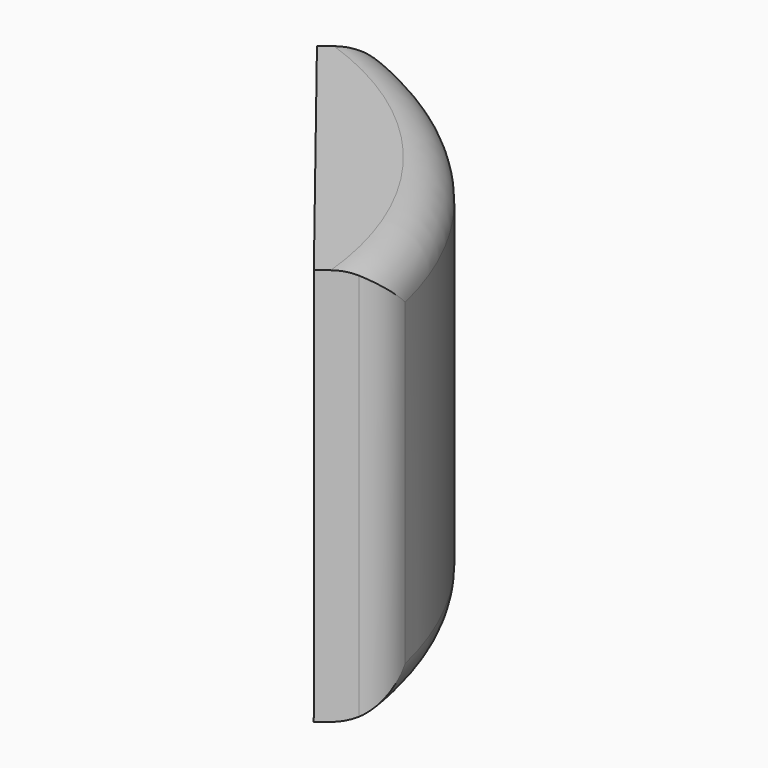
from build123d import *

# Parameters (mm, degrees)
F1_DEPTH     = 50.8
F2_W         = 48.4209248795
F2_H         = 50.8
F2_W_2       = 40.64
F2_H_2       = 40.64
F3_DEPTH     = 7.62
F4_T1_DEPTH  = 40.64
F4_T3_DEPTH  = 40.64
F4_T9_DEPTH  = 53.34
F4_T15_DEPTH = 53.34
F4_T24_DEPTH = 53.34
F4_T30_DEPTH = 53.34
F5_T1_DEPTH  = 40.64
F5_T6_DEPTH  = 17.2700101558
F5_S7_R      = 5.0800000001
F5_T8_DEPTH  = 13
F5_T12_DEPTH = 15.9109147238
F5_S13_R     = 5.0800000001
F5_T14_DEPTH = 12
F6_R         = 5.08


# Not quite as in the source:
# - a fillet or chamfer that OpenCascade refuses, or shapes differently, is made with other operations: its cross-section is extruded or revolved along the edge and cut away or added


with BuildPart() as f1:
    # F0 (on Top) → F1 (new body)
    with BuildSketch(Plane.XY):
        with BuildLine():
            Line((0, 38.0047485232), (30.0037506968, 0))
            ThreePointArc((30.0037506968, 0), (19.9032134253, 22.871851931), (0, 38.0047485232))
        make_face()
    extrude(amount=F1_DEPTH)

    # F2 (on face) → F3 (join)
    with BuildSketch(Plane(origin=(18.4835383706, 14.5922680406, 0), x_dir=(0.6196443123, -0.7848827468, 0), z_dir=(-0.7848827468, -0.6196443123, 0))):
        with Locations((-5.6188089735, 25.4)):
            Rectangle(F2_W, F2_H)
        with Locations((-6.2983566895, 25.7165116596)):
            Rectangle(F2_W_2, F2_H_2, mode=Mode.SUBTRACT)
    extrude(amount=F3_DEPTH)

    # F4: fillet of radius 5.08 on 3 edges, made by hand

    # F4_s2 → F4_t1 (cut)
    with BuildSketch(Plane(origin=(-16.4939133248, 20.8922889144, 0), x_dir=(0, 0, 1), z_dir=(0.6196443123, -0.7848827468, 0))):
        with BuildLine():
            ThreePointArc((46.0365116596, -21.0094262619), (47.5244092112, -17.4173238135), (51.1165116596, -15.9294262619))
            Line((51.1165116596, -15.9294262619), (46.0365116596, -15.9294262619))
            Line((46.0365116596, -15.9294262619), (46.0365116596, -21.0094262619))
        make_face()
    extrude(amount=F4_T1_DEPTH, mode=Mode.SUBTRACT)

    # F4_s4 → F4_t3 (cut)
    with BuildSketch(Plane.XY.offset(5.3965116596)):
        with BuildLine():
            ThreePointArc((25.1783677198, 2.0130255709), (23.2809557383, -1.3806253977), (24.3389564723, -5.1219718894))
            Line((24.3389564723, -5.1219718894), (21.1911633659, -1.1347675355))
            Line((21.1911633659, -1.1347675355), (25.1783677198, 2.0130255709))
        make_face()
        with BuildLine():
            ThreePointArc((-0.0039771311, 33.9106604018), (-3.7453236228, 32.8526596678), (-7.1389745914, 34.7500716493))
            Line((-7.1389745914, 34.7500716493), (-3.991181485, 30.7628672955))
            Line((-3.991181485, 30.7628672955), (-0.0039771311, 33.9106604018))
        make_face()
    extrude(amount=F4_T3_DEPTH, mode=Mode.SUBTRACT)


with BuildPart() as f4_tool7:
    # F4_s8 → F4_t9 (new body)
    with BuildSketch(Plane(origin=(-24.3633960907, 30.8602997991, 0), x_dir=(0, 0, 1), z_dir=(0.6196443123, -0.7848827468, 0))):
        with BuildLine():
            ThreePointArc((46.0365116596, -21.0094262619), (47.5244092112, -17.4173238135), (51.1165116596, -15.9294262619))
            Line((51.1165116596, -15.9294262619), (46.0365116596, -15.9294262619))
            Line((46.0365116596, -15.9294262619), (46.0365116596, -21.0094262619))
        make_face()
    extrude(amount=F4_T9_DEPTH)

    split(bisect_by=Plane(origin=(-16.4939133248, 20.8922889144, 0), x_dir=(0, 0, 1), z_dir=(-0.6196443123, 0.7848827468, 0)), keep=Keep.TOP)

    split(bisect_by=Plane.XY.offset(50.8), keep=Keep.BOTTOM)

    split(bisect_by=Plane(origin=(-18.4835383706, 23.4124804826, 0), x_dir=(0, 0, 1), z_dir=(0.6196443123, -0.7848827468, 0)), keep=Keep.TOP)


with BuildPart() as f4_tool13:
    # F4_s14 → F4_t15 (new body)
    with BuildSketch(Plane.XY.offset(5.3965116596)):
        with BuildLine():
            ThreePointArc((-0.0039771311, 33.9106604018), (-3.7453236228, 32.8526596678), (-7.1389745914, 34.7500716493))
            Line((-7.1389745914, 34.7500716493), (-3.991181485, 30.7628672955))
            Line((-3.991181485, 30.7628672955), (-0.0039771311, 33.9106604018))
        make_face()
    extrude(amount=F4_T15_DEPTH)

    split(bisect_by=Plane.XY.offset(46.0365116596), keep=Keep.TOP)

    split(bisect_by=Plane.XY.offset(50.8), keep=Keep.BOTTOM)

    split(bisect_by=Plane(origin=(-18.4835383706, 23.4124804826, 0), x_dir=(0, 0, 1), z_dir=(0.6196443123, -0.7848827468, 0)), keep=Keep.TOP)


with BuildPart() as f4_tool7_1:
    add(f4_tool7.part)

    # F4_t19: intersect F4_tool13
    add(f4_tool13.part, mode=Mode.INTERSECT)


with BuildPart() as f1_1:
    add(f1.part)

    # F4_t5: cut F4_tool7
    add(f4_tool7_1.part, mode=Mode.SUBTRACT)


with BuildPart() as f4_tool22:
    # F4_s23 → F4_t24 (new body)
    with BuildSketch(Plane(origin=(-16.4939133248, 20.8922889144, 0), x_dir=(0, 0, 1), z_dir=(0.6196443123, -0.7848827468, 0))):
        with BuildLine():
            ThreePointArc((46.0365116596, -21.0094262619), (47.5244092112, -17.4173238135), (51.1165116596, -15.9294262619))
            Line((51.1165116596, -15.9294262619), (46.0365116596, -15.9294262619))
            Line((46.0365116596, -15.9294262619), (46.0365116596, -21.0094262619))
        make_face()
    extrude(amount=F4_T24_DEPTH)

    split(bisect_by=Plane(origin=(8.6884315261, -11.0053459165, 0), x_dir=(0, 0, 1), z_dir=(0.6196443123, -0.7848827468, 0)), keep=Keep.TOP)

    split(bisect_by=Plane(origin=(11.5202123262, -14.5922680406, 0), x_dir=(0, 0, 1), z_dir=(-0.6196443123, 0.7848827468, 0)), keep=Keep.TOP)

    split(bisect_by=Plane.XY.offset(50.8), keep=Keep.BOTTOM)


with BuildPart() as f4_tool28:
    # F4_s29 → F4_t30 (new body)
    with BuildSketch(Plane.XY.offset(58.7365116596)):
        with BuildLine():
            ThreePointArc((25.1783677198, 2.0130255709), (23.2809557383, -1.3806253977), (24.3389564723, -5.1219718894))
            Line((24.3389564723, -5.1219718894), (21.1911633659, -1.1347675355))
            Line((21.1911633659, -1.1347675355), (25.1783677198, 2.0130255709))
        make_face()
    extrude(amount=-F4_T30_DEPTH)

    split(bisect_by=Plane.XY.offset(46.0365116596), keep=Keep.TOP)

    split(bisect_by=Plane(origin=(11.5202123262, -14.5922680406, 0), x_dir=(0, 0, 1), z_dir=(-0.6196443123, 0.7848827468, 0)), keep=Keep.TOP)

    split(bisect_by=Plane.XY.offset(50.8), keep=Keep.BOTTOM)


with BuildPart() as f4_tool22_1:
    add(f4_tool22.part)

    # F4_t34: intersect F4_tool28
    add(f4_tool28.part, mode=Mode.INTERSECT)


with BuildPart() as f1_2:
    add(f1_1.part)

    # F4_t20: cut F4_tool22
    add(f4_tool22_1.part, mode=Mode.SUBTRACT)

    # F5: fillet of radius 5.08 on 1 edges, made by hand

    # F5_s2 → F5_t1 (cut)
    with BuildSketch(Plane(origin=(8.6884315261, -11.0053459165, 0), x_dir=(0, 0, 1), z_dir=(-0.6196443123, 0.7848827468, 0))):
        with BuildLine():
            ThreePointArc((0.3165116596, 15.9294262619), (3.908614108, 17.4173238135), (5.3965116596, 21.0094262619))
            Line((5.3965116596, 21.0094262619), (5.3965116596, 15.9294262619))
            Line((5.3965116596, 15.9294262619), (0.3165116596, 15.9294262619))
        make_face()
    extrude(amount=F5_T1_DEPTH, mode=Mode.SUBTRACT)


with BuildPart() as f5_tool4:
    # F5_s5 → F5_t6 (new body)
    with BuildSketch(Plane(origin=(19.3896950922, -24.5602789253, 0), x_dir=(0, 0, 1), z_dir=(-0.6196443123, 0.7848827468, 0))):
        with BuildLine():
            ThreePointArc((0.3165116596, 15.9294262619), (3.908614108, 17.4173238135), (5.3965116596, 21.0094262619))
            Line((5.3965116596, 21.0094262619), (5.3965116596, 15.9294262619))
            Line((5.3965116596, 15.9294262619), (0.3165116596, 15.9294262619))
        make_face()
    extrude(amount=F5_T6_DEPTH)

    # F5_s7 → F5_t8 (cut, symmetric)
    with BuildSketch(Plane.XY.offset(2.9)):
        with Locations((28.3261608263, -1.974178783)):
            Circle(F5_S7_R)
    extrude(amount=F5_T8_DEPTH, both=True, mode=Mode.SUBTRACT)


with BuildPart() as f1_3:
    add(f1_2.part)

    # F5_t3: cut F5_tool4
    add(f5_tool4.part, mode=Mode.SUBTRACT)


with BuildPart() as f5_tool10:
    # F5_s11 → F5_t12 (new body)
    with BuildSketch(Plane(origin=(-26.3530211368, 33.3804913668, 0), x_dir=(0, 0, 1), z_dir=(0.6196443123, -0.7848827468, 0))):
        with BuildLine():
            ThreePointArc((0.3165116596, -15.9294262623), (3.908614108, -17.4173238139), (5.3965116596, -21.0094262623))
            Line((5.3965116596, -21.0094262623), (5.3965116596, -15.9294262623))
            Line((5.3965116596, -15.9294262623), (0.3165116596, -15.9294262623))
        make_face()
    extrude(amount=F5_T12_DEPTH)

    # F5_s13 → F5_t14 (cut, symmetric)
    with BuildSketch(Plane.XY.offset(2.9)):
        with Locations((-3.1517702375, 37.8978647558)):
            Circle(F5_S13_R)
    extrude(amount=F5_T14_DEPTH, both=True, mode=Mode.SUBTRACT)


with BuildPart() as f1_4:
    add(f1_3.part)

    # F5_t9: cut F5_tool10
    add(f5_tool10.part, mode=Mode.SUBTRACT)

    # F6
    f6_edges = [f1_4.edges().sort_by_distance(p)[0] for p in [
        (19.903213, 22.871852, 50.8),
        (30.003751, 0, 25.4),
        (19.903213, 22.871852, 0),
        (0, 38.004749, 25.4),
    ]]
    fillet(f6_edges, radius=F6_R)


solid = f1_4.part
